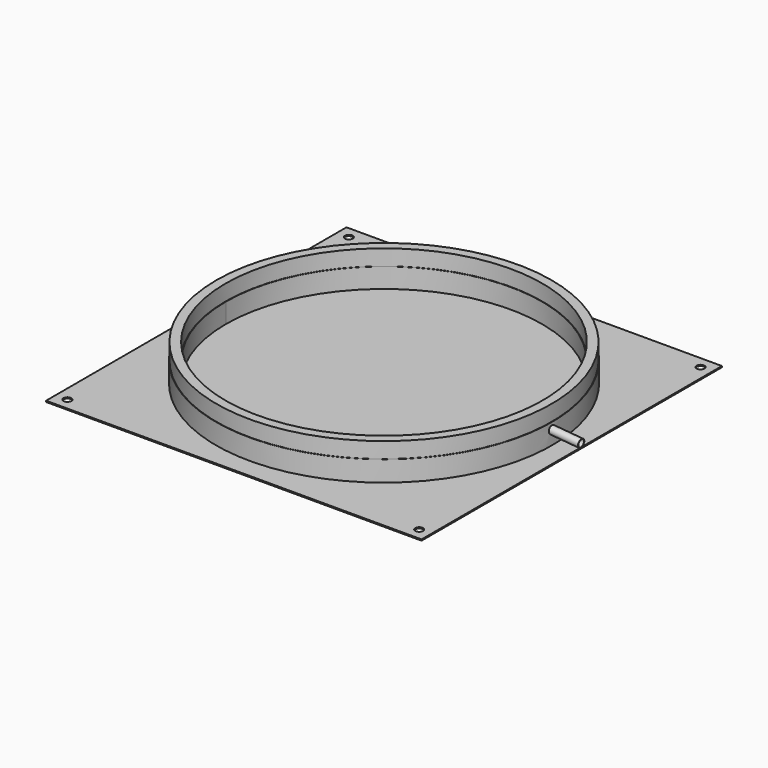
from build123d import *
from build123d import SkipClean  # not in build123d's __all__

# Parameters (mm, degrees)
F0_W     = 10
F0_H     = 3
F2_W     = 950
F2_H     = 950
F2_R     = 10
F3_DEPTH = 3
F6_R     = 9
F7_DEPTH = 120
F8_R     = 400
F9_DEPTH = 200


with BuildPart() as f1:
    # F0 (on Front) → F1 (revolve)
    with BuildSketch(Plane.XZ):
        Polygon((-425, 5), (-400, 5), (-400, 55), (-401, 55), (-401, 95), (-424, 95), (-424, 55), (-425, 55), align=None)
        Polygon((-10, 5), (-400, 5), (-425, 5), (-425, 2), (-10, 2), align=None)
        with Locations((-5, 3.5)):
            Rectangle(F0_W, F0_H)
    revolve(axis=Axis((0, 0, 187.9212413023), (0, 0, -1)))

    # F2 (on Top) → F3 (join)
    with BuildSketch(Plane.XY):
        Rectangle(F2_W, F2_H)
        with Locations((-445, -445)):
            Circle(F2_R, mode=Mode.SUBTRACT)
        with Locations((445, -445)):
            Circle(F2_R, mode=Mode.SUBTRACT)
        with Locations((-445, 445)):
            Circle(F2_R, mode=Mode.SUBTRACT)
        with Locations((445, 445)):
            Circle(F2_R, mode=Mode.SUBTRACT)
    extrude(amount=F3_DEPTH)

    # F4 (on Front) → F5 (revolve)
    with BuildSketch(Plane.XZ):
        Polygon((499.6194698092, 41.5098406888), (400, 50.2254149636), (399.9128442573, 49.2292202655), (499.5323140664, 40.5136459907), align=None)
    revolve(axis=Axis((512.7442754949, 0, 30.3233706049), (0.9961946981, 0, -0.0871557427)))

    # F6 (on face) → F7 (cut)
    with BuildSketch(Plane(origin=(492.2202445211, 0, -43.0636913536), x_dir=(0, 1, 0), z_dir=(0.9961946981, 0, -0.0871557427))):
        with Locations((0, 74.8965891952)):
            Circle(F6_R)
    extrude(amount=-F7_DEPTH, mode=Mode.SUBTRACT)

    # F8 (on face) → F9 (cut)
    with BuildSketch(Plane.XY.offset(5)):
        Circle(F8_R)
    with SkipClean():  # cleaning this boolean's faces spoils the solid; the shape is the same uncleaned
        extrude(amount=F9_DEPTH, mode=Mode.SUBTRACT)


solid = f1.part
